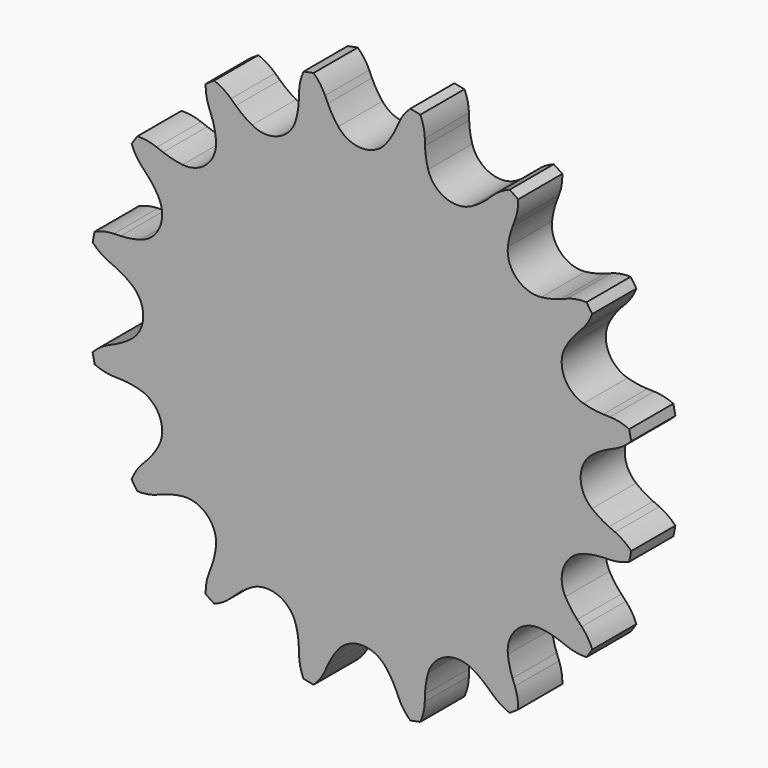
from build123d import *

# Parameters (mm, degrees)
F0_R            = 35.76066
F1_DEPTH        = 7.2136
F3_DEPTH        = 7.2146
F3_COPIES_COUNT = 16


# Not quite as in the source:
# - a pattern or mirror of a feature is missing from the dataset's text; its kind, count and spacing are read off the source's solid


with BuildPart() as f1:
    # F0 (on Front) → F1 (new body)
    with BuildSketch(Plane.XZ):
        Circle(F0_R)
    extrude(amount=-F1_DEPTH)

    # F2 (on face) → F3 (cut, through all)
    with BuildSketch(Plane.XZ):
        with BuildLine():
            Line((-4.8164154778, 33.0982711732), (-4.4568878106, 32.3001493474))
            ThreePointArc((-4.4568878106, 32.3001493474), (-3.8441959519, 31.1417538349), (-3.0902142758, 30.0699408338))
            ThreePointArc((-3.0902142758, 30.0699408338), (0, 28.5877), (3.0902142758, 30.0699408338))
            ThreePointArc((3.0902142758, 30.0699408338), (3.8441959519, 31.1417538349), (4.4568878106, 32.3001493474))
            Line((4.4568878106, 32.3001493474), (4.8164154778, 33.0982711732))
            ThreePointArc((4.8164154778, 33.0982711732), (5.4627291736, 34.2224644474), (6.3166306588, 35.198366166))
            ThreePointArc((6.3166306588, 35.198366166), (0, 35.76066), (-6.3166306588, 35.198366166))
            ThreePointArc((-6.3166306588, 35.198366166), (-5.4627291736, 34.2224644474), (-4.8164154778, 33.0982711732))
        make_face()
    f3 = extrude(amount=-F3_DEPTH, mode=Mode.SUBTRACT)

    # F3_copies: F3 ×16 about axis
    f3_copies_axis = Axis((0, 0, 0), (0, 1, 0))
    for i in range(1, F3_COPIES_COUNT):
        add(f3.rotate(f3_copies_axis, i * 360 / F3_COPIES_COUNT), mode=Mode.SUBTRACT)


solid = f1.part
